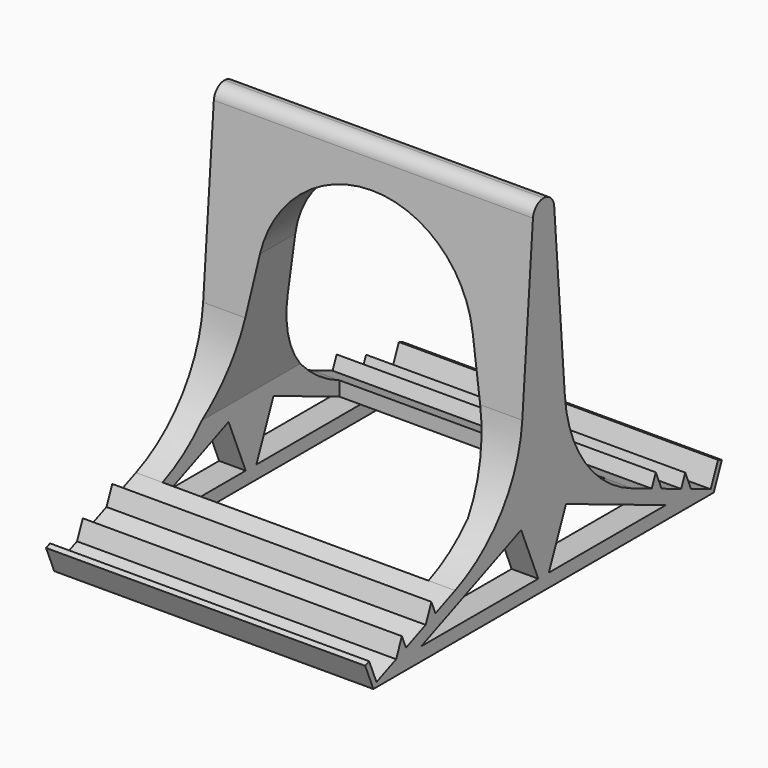
from build123d import *

# Parameters (mm, degrees)
F1_DEPTH   = 60
F3_DEPTH   = 25
F4_W       = 100
F4_H       = 41.5797430669
F5_DEPTH   = 30.001
F5_FACE_W  = 100
F5_FACE_H  = 5
F6_REACH   = 142.3730132293
F5_FACE1_W = 100
F5_FACE1_H = 5
F7_REACH   = 142.3730132293


with BuildPart() as f1:
    # F0 (on Right) → F1 (new body, symmetric)
    with BuildSketch(Plane.YZ):
        with BuildLine():
            Line((-80, 0), (0, 0))
            Line((0, 0), (80, 0))
            Line((80, 0), (83.8268343237, 9.2387953251))
            Line((83.8268343237, 9.2387953251), (81.9790752586, 10.0041621898))
            Line((81.9790752586, 10.0041621898), (78.5349243673, 1.6892463972))
            Line((78.5349243673, 1.6892463972), (69.2961290422, 5.5160807209))
            Line((69.2961290422, 5.5160807209), (66.5901485415, 12.0488955453))
            Line((66.5901485415, 12.0488955453), (64.6767313797, 7.4294978827))
            Line((64.6767313797, 7.4294978827), (55.4379360546, 11.2563322064))
            Line((55.4379360546, 11.2563322064), (52.7319555538, 17.7891470308))
            Line((52.7319555538, 17.7891470308), (50.818538392, 13.1697493682))
            Line((50.818538392, 13.1697493682), (41.5797430669, 16.9965836918))
            ThreePointArc((41.5797430669, 16.9965836918), (19.6436139822, 34.3018638475), (10, 60.5252730432))
            Line((10, 60.5252730432), (4.9851213736, 125.3854411629))
            ThreePointArc((4.9851213736, 125.3854411629), (3.3965272107, 128.6692782543), (0, 130))
            ThreePointArc((0, 130), (-3.3965272107, 128.6692782543), (-4.9851213736, 125.3854411629))
            Line((-4.9851213736, 125.3854411629), (-10, 60.5252730432))
            ThreePointArc((-10, 60.5252730432), (-19.6436139822, 34.3018638475), (-41.5797430669, 16.9965836918))
            Line((-41.5797430669, 16.9965836918), (-50.818538392, 13.1697493682))
            Line((-50.818538392, 13.1697493682), (-52.7319555538, 17.7891470308))
            Line((-52.7319555538, 17.7891470308), (-55.4379360546, 11.2563322064))
            Line((-55.4379360546, 11.2563322064), (-64.6767313797, 7.4294978827))
            Line((-64.6767313797, 7.4294978827), (-66.5901485415, 12.0488955453))
            Line((-66.5901485415, 12.0488955453), (-69.2961290422, 5.5160807209))
            Line((-69.2961290422, 5.5160807209), (-78.5349243673, 1.6892463972))
            Line((-78.5349243673, 1.6892463972), (-81.9790752586, 10.0041621898))
            Line((-81.9790752586, 10.0041621898), (-83.8268343237, 9.2387953251))
            Line((-83.8268343237, 9.2387953251), (-80, 0))
        make_face()
        Polygon((-10.5511115466, 24.437102688), (-2.5, 5), (-57.4764284691, 5), align=None, mode=Mode.SUBTRACT)
        Polygon((57.4764284691, 5), (2.5, 5), (10.5511115466, 24.437102688), align=None, mode=Mode.SUBTRACT)
    extrude(amount=F1_DEPTH, both=True)

    # F2 (on Front) → F3 (cut, symmetric)
    with BuildSketch(Plane.XZ):
        with BuildLine():
            ThreePointArc((0, 115.3854411629), (-25.9524271926, 106.0449266507), (-40, 82.3080484491))
            Line((-40, 82.3080484491), (-50, 30))
            Line((-50, 30), (0, 30))
            Line((0, 30), (50, 30))
            Line((50, 30), (40, 82.3080484491))
            ThreePointArc((40, 82.3080484491), (25.9524271926, 106.0449266507), (0, 115.3854411629))
        make_face()
    extrude(amount=F3_DEPTH, both=True, mode=Mode.SUBTRACT)

    # F4 (on face) → F5 (cut, through all)
    with BuildSketch(Plane.XY.offset(30)):
        with Locations((0, 20.7898715334)):
            Rectangle(F4_W, F4_H)
        with Locations((0, -20.7898715334)):
            Rectangle(F4_W, F4_H)
    extrude(amount=-F5_DEPTH, mode=Mode.SUBTRACT)

    f6_end = Plane(origin=(0, 43.7688782858, 10.6778531928), x_dir=(0, -0.9238795325, 0.3826834324), z_dir=(0, -0.3826834324, -0.9238795325))
    # F5_face (on face) → F6 (cut, up to a plane its end follows)
    with BuildSketch(Plane(origin=(0, 41.5797430669, 2.5), x_dir=(1, 0, 0), z_dir=(0, -1, 0))):
        Rectangle(F5_FACE_W, F5_FACE_H)
    f6_long = extrude(amount=-F6_REACH, mode=Mode.PRIVATE)
    add(split(f6_long, bisect_by=f6_end, keep=Keep.TOP, mode=Mode.PRIVATE), mode=Mode.SUBTRACT)

    f7_end = Plane(origin=(0, -43.7688782858, 10.6778531928), x_dir=(0, -0.9238795325, -0.3826834324), z_dir=(0, 0.3826834324, -0.9238795325))
    # F5_face1 (on face) → F7 (cut, up to a plane its end follows)
    with BuildSketch(Plane(origin=(0, -41.5797430669, 2.5), x_dir=(-1, 0, 0), z_dir=(0, 1, 0))):
        Rectangle(F5_FACE1_W, F5_FACE1_H)
    f7_long = extrude(amount=-F7_REACH, mode=Mode.PRIVATE)
    add(split(f7_long, bisect_by=f7_end, keep=Keep.TOP, mode=Mode.PRIVATE), mode=Mode.SUBTRACT)


solid = f1.part
